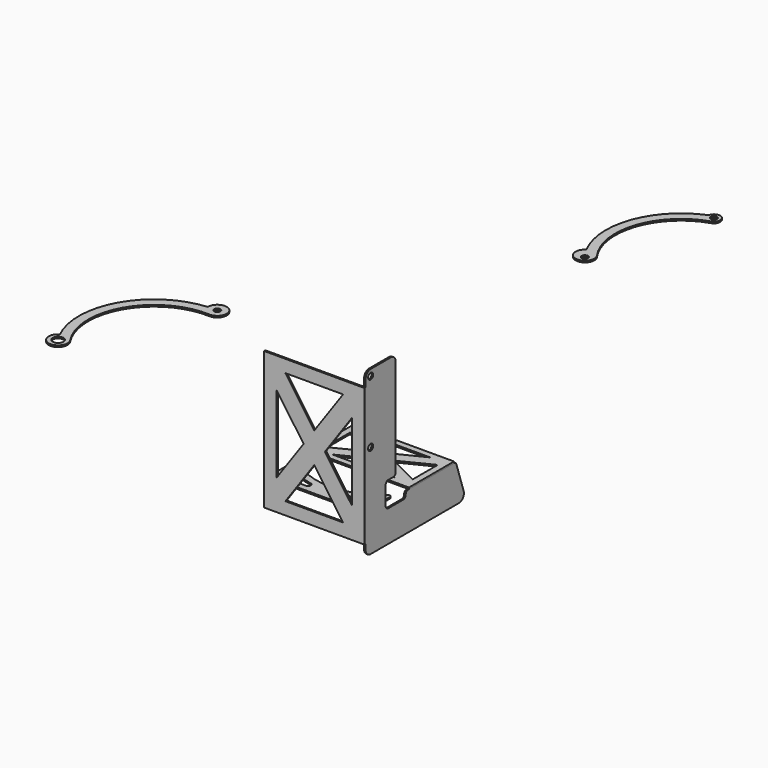
from build123d import *

# Parameters (mm, degrees)
F0_R      = 6.35
F1_DEPTH  = 3.175
F2_R      = 12.7
F3_R      = 6.34999
F4_W      = 203.2
F4_H      = 114.3
F5_DEPTH  = 3.175
F6_W      = 203.2
F6_H      = 279.4
F7_DEPTH  = 3.175
F10_DEPTH = 3.175
F11_R     = 4.445
F12_R     = 12.7
F13_R     = 10.795
F13_R_2   = 6.35
F14_DEPTH = 3.175
F15_R     = 6.35
F16_DEPTH = 3.175


# Not quite as in the source:
# - a fillet or chamfer is up to 0.001 mm smaller than in the source, because OpenCascade refuses the exact size


with BuildPart() as f1:
    # F0 (on Right) → F1 (new body)
    with BuildSketch(Plane.YZ):
        Polygon((25.4, -12.7), (0, -12.7), (-25.4, -12.7), (-25.4, 38.1), (0, 38.1), (0, 254), (-76.2, 254), (-76.2, -76.2), (177.8, -76.2), (152.4, 0), (25.4, 0), align=None)
        with Locations((-63.5, 114.3)):
            Circle(F0_R, mode=Mode.SUBTRACT)
        with Locations((-63.5, 241.3)):
            Circle(F0_R, mode=Mode.SUBTRACT)
    extrude(amount=F1_DEPTH)

    # F2
    f2_edges = [f1.edges().sort_by_distance(p)[0] for p in [
        (1.5875, -76.2, 254),
        (1.5875, 0, 254),
    ]]
    fillet(f2_edges, radius=F2_R)

    # F3 (radius 6.35 in the source; OpenCascade refuses exactly that, so slightly less here)
    f3_edges = [f1.edges().sort_by_distance(p)[0] for p in [
        (1.5875, 152.4, 0),
        (1.5875, 25.4, 0),
        (1.5875, 25.4, -12.7),
        (1.5875, -25.4, 38.1),
        (1.5875, 0, 38.1),
        (1.5875, -25.4, -12.7),
    ]]
    fillet(f3_edges, radius=F3_R)

    # F12
    f12_edges = [f1.edges().sort_by_distance(p)[0] for p in [
        (1.5875, -76.2, -76.2),
        (1.5875, 177.8, -76.2),
    ]]
    fillet(f12_edges, radius=F12_R)


with BuildPart() as f5:
    # F4 (on face) → F5 (new body)
    with BuildSketch(Plane.XY):
        with Locations((-98.425, 90.6731789526)):
            Rectangle(F4_W, F4_H)
        Polygon((-34.925, 46.2296610243), (-161.925, 46.2296610243), (-98.425, 77.9795901259), align=None, mode=Mode.SUBTRACT)
        Polygon((-187.325, 58.9296610243), (-187.325, 122.4294908681), (-123.8250283594, 90.6795759462), align=None, mode=Mode.SUBTRACT)
        Polygon((-73.0249716406, 90.6795759462), (-9.525, 122.4294908681), (-9.525, 58.9296610243), align=None, mode=Mode.SUBTRACT)
        Polygon((-98.425, 103.3795617665), (-161.9253403131, 135.1296610243), (-34.9246596869, 135.1296610243), align=None, mode=Mode.SUBTRACT)
    extrude(amount=F5_DEPTH)


with BuildPart() as f7:
    # F6 (on face) → F7 (new body)
    with BuildSketch(Plane.XZ.offset(76.2)):
        with Locations((-98.425, 101.6)):
            Rectangle(F6_W, F6_H)
        Polygon((-98.425, 70.7571428571), (-40.005, -12.7), (-156.845, -12.7), align=None, mode=Mode.SUBTRACT)
        Polygon((-76.835, 101.6), (-22.225, 179.6142857143), (-22.225, 23.5857142857), align=None, mode=Mode.SUBTRACT)
        Polygon((-174.625, 23.5857142857), (-174.625, 179.6142857143), (-120.015, 101.6), align=None, mode=Mode.SUBTRACT)
        Polygon((-98.425, 132.4428571429), (-156.845, 215.9), (-40.005, 215.9), align=None, mode=Mode.SUBTRACT)
    extrude(amount=F7_DEPTH)


with BuildPart() as f7_1:
    # F8: moved
    add(f7.part.moved(Location((0, 0, -14.732))))


with BuildPart() as f10:
    # F9 (on Top) → F10 (new body)
    with BuildSketch(Plane.XY):
        with BuildLine():
            ThreePointArc((0, 0), (-97.155, -42.0092726381), (-194.31, 0))
            Line((-194.31, 0), (-194.31, -76.2))
            Line((-194.31, -76.2), (0, -76.2))
            Line((0, -76.2), (0, 0))
        make_face()
        with BuildLine():
            Line((-122.555, -63.5), (-181.61, -63.5))
            Line((-181.61, -63.5), (-181.61, -28.874717996))
            ThreePointArc((-181.61, -28.874717996), (-153.4504018439, -44.4838948062), (-122.555, -53.5438900549))
            Line((-122.555, -53.5438900549), (-122.555, -63.5))
        make_face(mode=Mode.SUBTRACT)
        with BuildLine():
            Line((-12.7, -28.874717996), (-12.7, -63.5))
            Line((-12.7, -63.5), (-71.755, -63.5))
            Line((-71.755, -63.5), (-71.755, -53.5438900549))
            ThreePointArc((-71.755, -53.5438900549), (-40.8595981561, -44.4838948062), (-12.7, -28.874717996))
        make_face(mode=Mode.SUBTRACT)
    extrude(amount=F10_DEPTH)

    # F11
    f11_edges = [f10.edges().sort_by_distance(p)[0] for p in [
        (-122.555, -63.5, 1.5875),
        (-122.555, -53.54389, 1.5875),
        (-181.61, -63.5, 1.5875),
        (-181.61, -28.874718, 1.5875),
        (-12.7, -63.5, 1.5875),
        (-71.755, -63.5, 1.5875),
        (-71.755, -53.54389, 1.5875),
        (-12.7, -28.874718, 1.5875),
        (-194.31, 0, 1.5875),
        (0, 0, 1.5875),
    ]]
    fillet(f11_edges, radius=F11_R)


with BuildPart() as f14:
    # F13 (on Top) → F14 (new body)
    with BuildSketch(Plane.XY):
        with BuildLine():
            ThreePointArc((-632.1968888271, 318.0701347804), (-752.3858015786, 241.1343877568), (-756.2063521379, 98.4813565521))
            ThreePointArc((-756.2063521379, 98.4813565521), (-751.0570291306, 63.4352752545), (-730.811212931, 92.5015833821))
            ThreePointArc((-730.811212931, 92.5015833821), (-735.8008176206, 231.7641386358), (-613.9695684644, 299.4110319849))
            ThreePointArc((-613.9695684644, 299.4110319849), (-599.523415155, 331.7552091602), (-632.1968888271, 318.0701347804))
        make_face()
        with Locations((-746.6907536235, 81.9781482303)):
            Circle(F13_R, mode=Mode.SUBTRACT)
        with Locations((-613.1505463981, 318.4434176172)):
            Circle(F13_R_2, mode=Mode.SUBTRACT)
    extrude(amount=F14_DEPTH)


with BuildPart() as f16:
    # F15 (on Top) → F16 (new body)
    with BuildSketch(Plane.XY):
        with BuildLine():
            ThreePointArc((-261.2709873869, 840.5799733082), (-278.8922283797, 959.7951557271), (-193.2070800325, 1044.5348937844))
            ThreePointArc((-193.2070800325, 1044.5348937844), (-188.7425781177, 1066.1939476514), (-209.5987572531, 1058.8409765764))
            ThreePointArc((-209.5987572532, 1058.8409765764), (-295.6765455954, 969.5204824254), (-286.8307241935, 845.7897757879))
            ThreePointArc((-286.8307241935, 845.7897757879), (-280.6286867095, 810.9134731448), (-261.2709873869, 840.5799733082))
        make_face()
        with Locations((-273.0500046197, 824.472849402)):
            Circle(F15_R, mode=Mode.SUBTRACT)
        with Locations((-197.0934681671, 1056.6256335165)):
            Circle(F15_R, mode=Mode.SUBTRACT)
    extrude(amount=F16_DEPTH)


solid = Compound([f1.part, f5.part, f7_1.part, f10.part, f14.part, f16.part])
